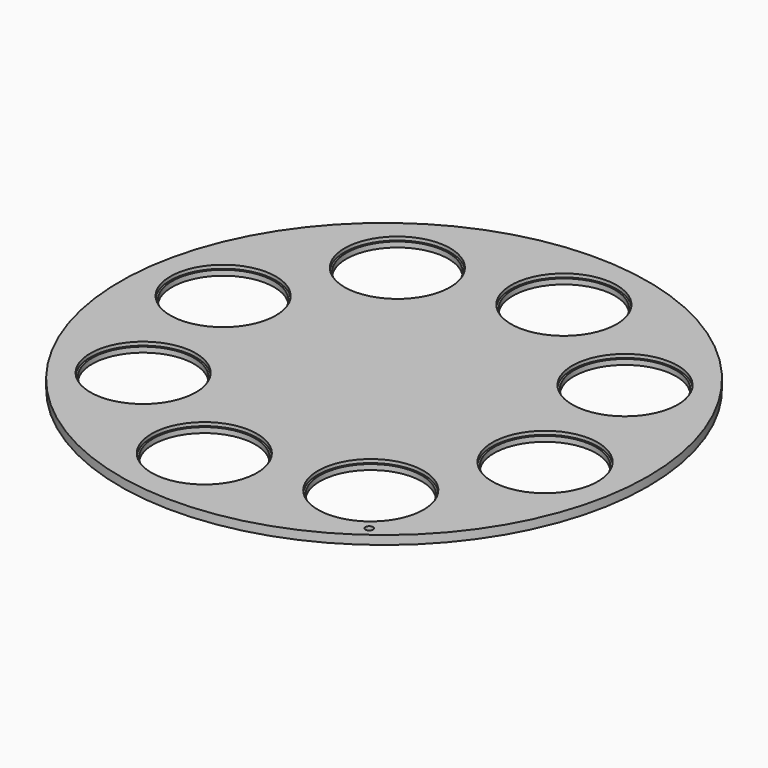
from build123d import *

# Parameters (mm, degrees)
F0_R            = 150
F1_DEPTH        = 2.5
F2_R            = 29
F3_DEPTH        = 5.001
F3_COPIES_COUNT = 8
F2_R_2          = 30
F4_DEPTH        = 2
F4_COPIES_COUNT = 8
F5_R            = 2.0850492766
F6_DEPTH        = 5.001


# Not quite as in the source:
# - a pattern or mirror of a feature is missing from the dataset's text; its kind, count and spacing are read off the source's solid


with BuildPart() as f1:
    # F0 (on Top) → F1 (new body, symmetric)
    with BuildSketch(Plane.XY):
        Circle(F0_R)
    extrude(amount=F1_DEPTH, both=True)

    # F2 (on face) → F3 (cut, through all)
    with BuildSketch(Plane.XY.offset(2.5)):
        with Locations((17.6781384332, 105.6203827018)):
            Circle(F2_R)
    f3 = extrude(amount=-F3_DEPTH, mode=Mode.SUBTRACT)

    # F3_copies: F3 ×8 about axis
    f3_copies_axis = Axis((0, 0, 0), (0, 0, 1))
    for i in range(1, F3_COPIES_COUNT):
        add(f3.rotate(f3_copies_axis, i * 360 / F3_COPIES_COUNT), mode=Mode.SUBTRACT)

    # F2 (on face) → F4 (cut)
    with BuildSketch(Plane.XY.offset(2.5)):
        with Locations((17.6781384332, 105.6203827018)):
            Circle(F2_R_2)
        with Locations((17.6781384332, 105.6203827018)):
            Circle(F2_R, mode=Mode.SUBTRACT)
    f4 = extrude(amount=-F4_DEPTH, mode=Mode.SUBTRACT)

    # F4_copies: F4 ×8 about axis
    f4_copies_axis = Axis((0, 0, 0), (0, 0, 1))
    for i in range(1, F4_COPIES_COUNT):
        add(f4.rotate(f4_copies_axis, i * 360 / F4_COPIES_COUNT), mode=Mode.SUBTRACT)

    # F5 (on face) → F6 (cut, through all)
    with BuildSketch(Plane.XY.offset(2.5)):
        with Locations((84.5384001732, -116.1978319287)):
            Circle(F5_R)
    extrude(amount=-F6_DEPTH, mode=Mode.SUBTRACT)


solid = f1.part
